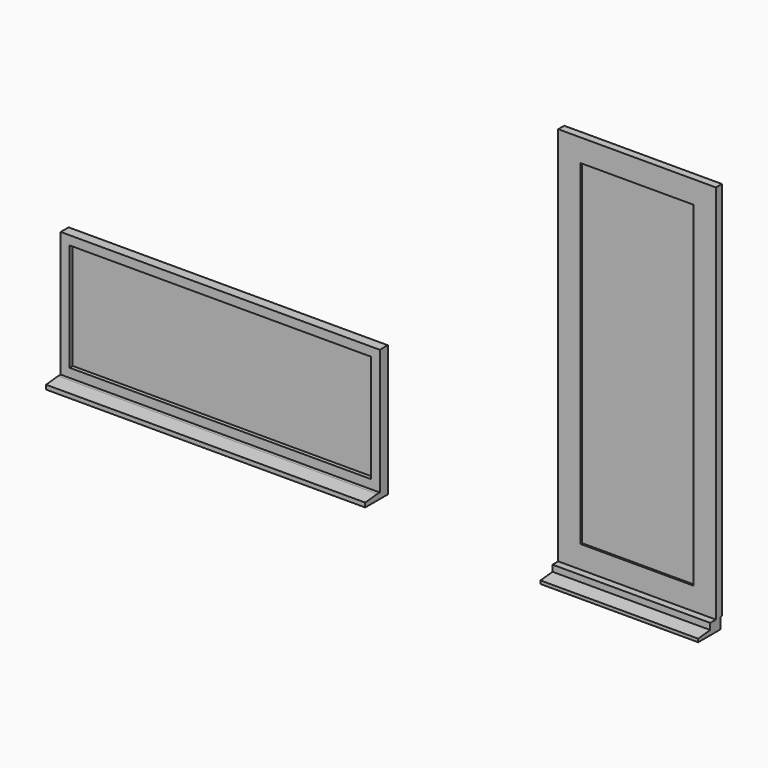
from build123d import *

# Parameters (mm, degrees)
F0_W      = 150
F0_H      = 31
F1_DEPTH  = 1700
F3_W      = 53
F3_H      = 47.5
F6_W      = 1605
F6_H      = 574
F7_DEPTH  = 22
F10_DEPTH = 840
F12_W     = 840
F12_H     = 2026.5
F12_W_2   = 600
F12_H_2   = 1786.5
F13_DEPTH = 40
F15_W     = 600
F15_H     = 1786.5
F16_DEPTH = 20
F17_SIZE2 = 8
F17_SIZE  = 80
F18_SIZE2 = 79.99999
F18_SIZE  = 7.99999


# Not quite as in the source:
# - a fillet or chamfer is up to 0.001 mm smaller than in the source, because OpenCascade refuses the exact size


with BuildPart() as f1:
    # F0 (on Right) → F1 (new body)
    with BuildSketch(Plane.YZ):
        with Locations((8.0352395773, 15.5)):
            Rectangle(F0_W, F0_H)
    extrude(amount=-F1_DEPTH)

    # F4: sweep along a path in F2
    with BuildLine(Plane(origin=(0, 83.0352395773, 0), x_dir=(-1, 0, 0), z_dir=(0, 1, 0))) as f4_path:
        Line((0, 31), (1700, 31))
        Line((1700, 31), (1700, 700))
        Line((1700, 700), (0, 700))
        Line((0, 700), (0, 31))
    # F3 (on Right) → F4 (sweep)
    with BuildSketch(Plane.YZ):
        with Locations((56.5352395773, 54.75)):
            Rectangle(F3_W, F3_H)
    sweep(path=f4_path.line, transition=Transition.RIGHT)

    # F17
    f17_edges = [f1.edges().sort_by_distance(p)[0] for p in [
        (-850, -66.96476, 31),
    ]]
    f17_side = f1.faces().sort_by_distance((-850, -18.46476, 31))[0]
    chamfer(f17_edges, length=F17_SIZE, length2=F17_SIZE2, reference=f17_side)


with BuildPart() as f7:
    # F6 (on offset) → F7 (new body)
    with BuildSketch(Plane(origin=(0, 73.0352395773, 0), x_dir=(-1, 0, 0), z_dir=(0, 1, 0))):
        with Locations((850, 365.5)):
            Rectangle(F6_W, F6_H)
    extrude(amount=-F7_DEPTH)


with BuildPart() as f10:
    # F9 (on offset) → F10 (new body)
    with BuildSketch(Plane.YZ.offset(1000)):
        Polygon((-150, 0), (0, 0), (0, 25), (0, 58.5), (-70, 58.5), (-70, 25), (-150, 25), align=None)
    extrude(amount=F10_DEPTH)

    # F12 (on offset) → F13 (join)
    with BuildSketch(Plane(origin=(0, 8, 0), x_dir=(-1, 0, 0), z_dir=(0, 1, 0))):
        with Locations((-1420, 1071.75)):
            Rectangle(F12_W, F12_H)
        with Locations((-1420, 1071.75)):
            Rectangle(F12_W_2, F12_H_2, mode=Mode.SUBTRACT)
    extrude(amount=-F13_DEPTH)

    # F18 (size 8 and 80 in the source; OpenCascade refuses exactly that, so slightly less here)
    f18_edges = [f10.edges().sort_by_distance(p)[0] for p in [
        (1420, -150, 25),
    ]]
    f18_side = f10.faces().sort_by_distance((1420, -150, 12.5))[0]
    chamfer(f18_edges, length=F18_SIZE, length2=F18_SIZE2, reference=f18_side)


with BuildPart() as f16:
    # F15 (on offset) → F16 (new body)
    with BuildSketch(Plane(origin=(0, -2, 0), x_dir=(-1, 0, 0), z_dir=(0, 1, 0))):
        with Locations((-1420, 1071.75)):
            Rectangle(F15_W, F15_H)
    extrude(amount=-F16_DEPTH)


solid = Compound([f1.part, f7.part, f10.part, f16.part])
